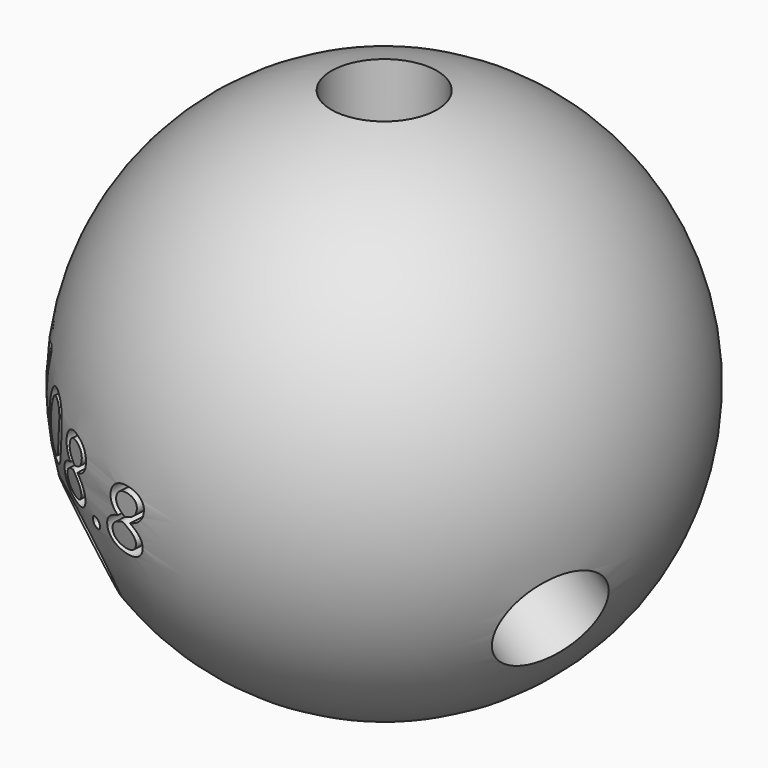
from build123d import *

# Parameters (mm, degrees)
F4_R          = 3.175
F5_DEPTH      = 50.8
F7_ANGLE      = 113.4
F8_ANGLE      = 108.2
F9_ANGLE      = 108.8
F11_TEXT_SIZE = 5.6107431495
F12_DEPTH     = 25.4
F14_TEXT_SIZE = 5.2600736833
F15_DEPTH     = 25.4


# Not quite as in the source:
# - Text() gives the source's letters only with a copy of the font that has no kerning and outlines rounded to 1/6400 em; it was checked with that copy


with BuildPart() as f2:
    # F0 (on Front) → F2 (revolve)
    with BuildSketch(Plane.XZ):
        with BuildLine():
            Line((0, -15.875), (0, 15.875))
            ThreePointArc((0, 15.875), (-15.875, 0), (0, -15.875))
        make_face()
    revolve(axis=Axis((0, 0, 0), (0, 0, 1)))

    # F11 (on offset) → F12 (cut)
    with BuildSketch(Plane(origin=(0, 32.6353544893, -14.122578991), x_dir=(-1, 0, 0), z_dir=(0, 0.9177546257, -0.3971478906))):
        with Locations((-7.3151026372, 3.3607012592)):
            Text('113.4', F11_TEXT_SIZE, font='Open Sans', text_align=(TextAlign.LEFT, TextAlign.BOTTOM))
    extrude(amount=-F12_DEPTH, mode=Mode.SUBTRACT)

    # F14 (on offset) → F15 (cut)
    with BuildSketch(Plane(origin=(-19.6404466176, -26.0637529782, -14.122578991), x_dir=(0.8336331633, -0.485612461, -0.2631278905), z_dir=(-0.5523185213, -0.7329514336, -0.3971478906))):
        with Locations((-6.6908088629, 3.5978914239)):
            Text('108.8', F14_TEXT_SIZE, font='Open Sans', text_align=(TextAlign.LEFT, TextAlign.BOTTOM))
    extrude(amount=-F15_DEPTH, mode=Mode.SUBTRACT)


with BuildPart() as f5:
    # F4 (on offset) → F5 (new body)
    with BuildSketch(Plane.XY.offset(10.16)):
        Circle(F4_R)
    extrude(amount=F5_DEPTH)


with BuildPart() as f7_1:
    # F7: copy of F5
    add(f5.part.rotate(Axis((-36.3165959716, 0, 0), (-1, 0, 0)), F7_ANGLE))


with BuildPart() as f8_1:
    # F8: copy of F7_1
    add(f7_1.part.rotate(Axis((0, 0, -29.0343631059), (0, 0, -1)), F8_ANGLE))


with BuildPart() as f9_1:
    # F9: copy of F8_1
    add(f8_1.part.rotate(Axis((0, 0, -29.0343631059), (0, 0, -1)), F9_ANGLE))


with BuildPart() as f2_1:
    add(f2.part)

    # F16: cut F5, F7_1, F9_1, F8_1
    add(f5.part, mode=Mode.SUBTRACT)
    add(f7_1.part, mode=Mode.SUBTRACT)
    add(f9_1.part, mode=Mode.SUBTRACT)
    add(f8_1.part, mode=Mode.SUBTRACT)


solid = f2_1.part
